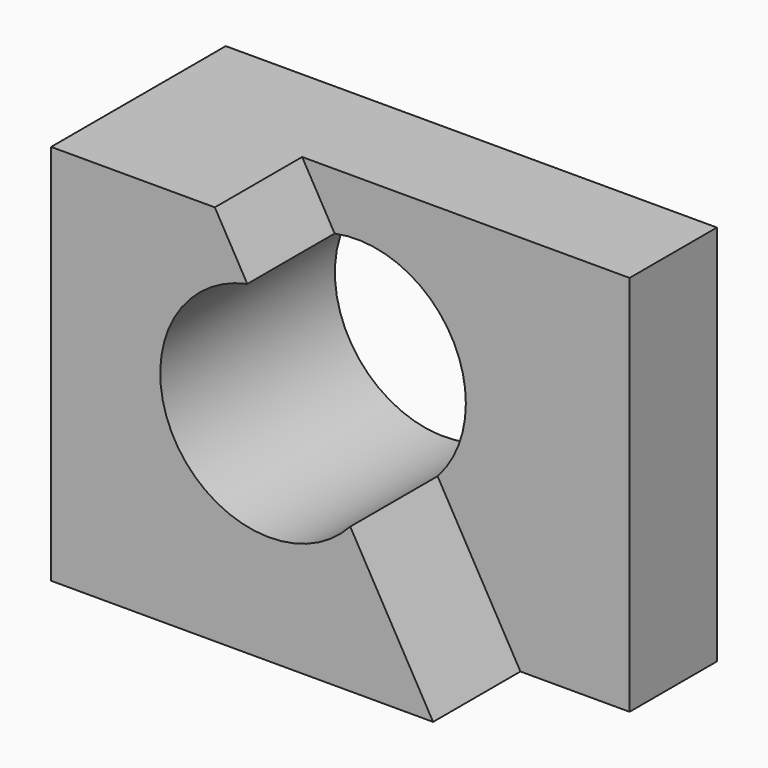
from build123d import *

# Parameters (mm, degrees)
F0_W     = 57.15
F0_H     = 44.45
F1_DEPTH = 25.4
F2_R     = 12.7
F3_DEPTH = 25.4
F5_DEPTH = 12.7


with BuildPart() as f1:
    # F0 (on Front) → F1 (new body)
    with BuildSketch(Plane.XZ):
        with Locations((28.575, 22.225)):
            Rectangle(F0_W, F0_H)
    extrude(amount=F1_DEPTH)

    # F2 (on face) → F3 (cut)
    with BuildSketch(Plane.XZ.offset(25.4)):
        with Locations((25.4, 25.4)):
            Circle(F2_R)
    extrude(amount=-F3_DEPTH, mode=Mode.SUBTRACT)

    # F4 (on face) → F5 (cut)
    with BuildSketch(Plane.XZ.offset(25.4)):
        with BuildLine():
            Line((57.15, 44.45), (19.05, 44.45))
            Line((19.05, 44.45), (22.8288518953, 37.8370091832))
            ThreePointArc((22.8288518953, 37.8370091832), (33.4198634362, 35.2474255755), (38.1, 25.4))
            ThreePointArc((38.1, 25.4), (37.2488826998, 20.8290068075), (34.8096096432, 16.8706831245))
            Line((34.8096096432, 16.8706831245), (44.45, 0))
            Line((44.45, 0), (57.15, 0))
            Line((57.15, 0), (57.15, 44.45))
        make_face()
    extrude(amount=-F5_DEPTH, mode=Mode.SUBTRACT)


solid = f1.part
